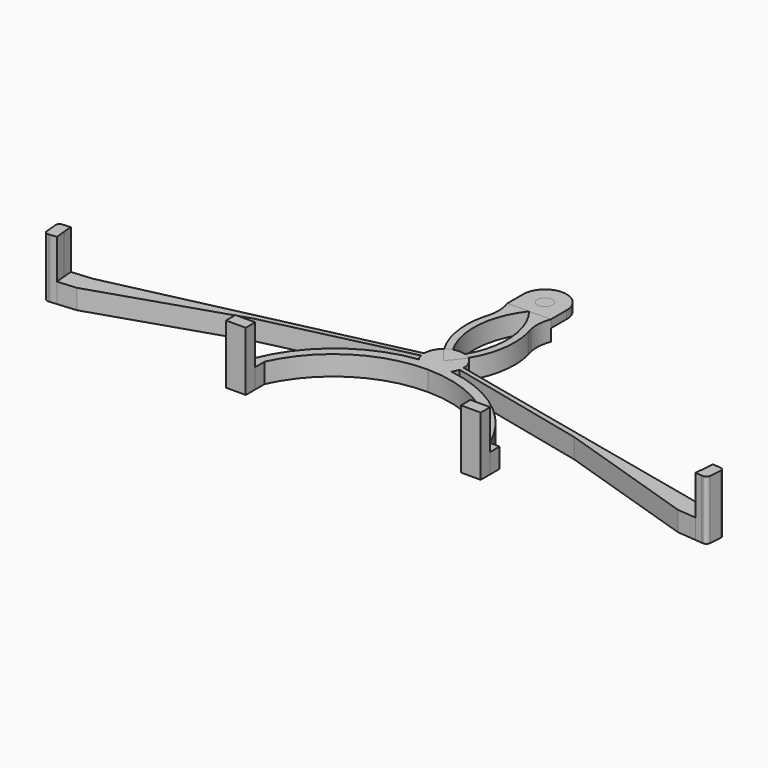
from build123d import *

# Parameters (mm, degrees)
F1_DEPTH = 15
F2_DEPTH = 5
F0_W     = 2.5
F0_H     = 3
F3_DEPTH = 5
F0_R     = 1.9
F4_DEPTH = 5
F5_DEPTH = 5
F6_DEPTH = 3


with BuildPart() as f1:
    # F0 (on Top) → F1 (new body)
    with BuildSketch(Plane.XY):
        with BuildLine():
            Line((-82.5, -21.5863350366), (-82.5, -16.5665013937))
            Line((-82.5, -16.5665013937), (-83.3699967597, -16.6440687753))
            ThreePointArc((-83.3699967597, -16.6440687753), (-84.0295454731, -16.9887980437), (-84.2521564375, -17.6989298148))
            Line((-84.2521564375, -17.6989298148), (-83.9808279356, -20.7421538184))
            ThreePointArc((-83.9808279356, -20.7421538184), (-83.6360986672, -21.4017025318), (-82.9259668961, -21.6243134962))
            Line((-82.9259668961, -21.6243134962), (-82.5, -21.5863350366))
        make_face()
        Polygon((-81.128345354, -18.9541238984), (-81.3503602858, -16.464001538), (-82.5, -16.5665013937), (-82.5, -21.5863350366), (-80.9063304222, -21.4442462589), align=None)
    extrude(amount=F1_DEPTH)


with BuildPart() as f1b:
    # F0 (on Top) → F1, piece 2 (new body)
    with BuildSketch(Plane.XY):
        with BuildLine():
            Line((83.3699963437, -16.6440687785), (82.5, -16.5665014329))
            Line((82.5, -16.5665014329), (82.5, -21.5863350764))
            Line((82.5, -21.5863350764), (82.9259664737, -21.6243134988))
            ThreePointArc((82.9259664737, -21.6243134988), (83.6360982451, -21.4017025353), (83.9808275143, -20.7421538224))
            Line((83.9808275143, -20.7421538224), (84.2521560202, -17.6989298191))
            ThreePointArc((84.2521560202, -17.6989298191), (84.0295450567, -16.9887980477), (83.3699963437, -16.6440687785))
        make_face()
        Polygon((82.5, -16.5665014329), (81.3503598701, -16.4640015386), (81.128344935, -18.9541238987), (80.90633, -21.4442462589), (82.5, -21.5863350764), align=None)
    extrude(amount=F1_DEPTH)


with BuildPart() as f1c:
    # F0 (on Top) → F1, piece 3 (new body)
    with BuildSketch(Plane.XY):
        Polygon((31.6213203436, -24.8786796564), (29.1213203436, -24.8786796564), (26.6213203436, -24.8786796564), (26.6213203436, -27.8786796564), (31.6213203436, -27.8786796564), align=None)
    extrude(amount=F1_DEPTH)


with BuildPart() as f1d:
    # F0 (on Top) → F1, piece 4 (new body)
    with BuildSketch(Plane.XY):
        Polygon((-29.8816396128, -25.5282291926), (-32.3816343716, -25.5231100091), (-32.3816343716, -28.5231100091), (-27.381644854, -28.5231100091), (-27.381644854, -25.5333483762), align=None)
    extrude(amount=F1_DEPTH)


with BuildPart() as f2:
    # F0 (on Top) → F2 (new body)
    with BuildSketch(Plane.XY):
        with BuildLine():
            Line((-2.1337940049, 27), (-5.5, 27))
            ThreePointArc((-5.5, 27), (-4.8940649659, 24.1020455305), (-5.1039532491, 21.1488702426))
            ThreePointArc((-5.1039532491, 21.1488702426), (-3.850388388, 24.1919569907), (-2.1337940049, 27))
        make_face()
        with BuildLine():
            Line((0, 27), (-2.1337940049, 27))
            ThreePointArc((-2.1337940049, 27), (-3.850388388, 24.1919569907), (-5.1039532491, 21.1488702426))
            ThreePointArc((-5.1039532491, 21.1488702426), (-5.278437838, 20.4458640026), (-5.5, 19.7562460986))
            ThreePointArc((-5.5, 19.7562460986), (-5.8710956961, 11.6043025747), (-3.0863215981, 3.9337792252))
            ThreePointArc((-3.0863215981, 3.9337792252), (-2.3467663768, 4.4150523862), (-1.5341266757, 4.7588291988))
            ThreePointArc((-1.5341266757, 4.7588291988), (-4.1864100938, 16.1152704866), (0, 27))
        make_face()
    extrude(amount=F2_DEPTH)


with BuildPart() as f2b:
    # F0 (on Top) → F2, piece 2 (new body)
    with BuildSketch(Plane.XY):
        with BuildLine():
            Line((2.1337940049, 27), (0, 27))
            ThreePointArc((0, 27), (4.1765920633, 16.1147529743), (1.5306162106, 4.7599594553))
            ThreePointArc((1.5306162106, 4.7599594553), (2.3451379758, 4.4159175575), (3.0863215981, 3.9337792252))
            ThreePointArc((3.0863215981, 3.9337792252), (5.8710956961, 11.6043025747), (5.5, 19.7562460986))
            ThreePointArc((5.5, 19.7562460986), (5.2493596136, 20.5144731098), (5.0579844363, 21.289782303))
            ThreePointArc((5.0579844363, 21.289782303), (3.8167255549, 24.2579809722), (2.1337940049, 27))
        make_face()
        with BuildLine():
            Line((5.5, 27), (2.1337940049, 27))
            ThreePointArc((2.1337940049, 27), (3.8167255549, 24.2579809722), (5.0579844363, 21.289782303))
            ThreePointArc((5.0579844363, 21.289782303), (4.8757325261, 24.1761066094), (5.5, 27))
        make_face()
    extrude(amount=F2_DEPTH)


with BuildPart() as f2c:
    # F0 (on Top) → F2, piece 3 (new body)
    with BuildSketch(Plane.XY):
        with BuildLine():
            ThreePointArc((0, 0), (-1.6614515986, 1.8740823074), (-3.0863215981, 3.9337792252))
            ThreePointArc((-3.0863215981, 3.9337792252), (-4.4961988385, 2.1872805043), (-5, 0))
            Line((-5, 0), (0, 0))
        make_face()
        with BuildLine():
            ThreePointArc((5, 0), (4.4961988385, 2.1872805043), (3.0863215981, 3.9337792252))
            ThreePointArc((3.0863215981, 3.9337792252), (1.6614515986, 1.8740823074), (0, 0))
            Line((0, 0), (5, 0))
        make_face()
        with BuildLine():
            Line((0, 0), (-5, 0))
            ThreePointArc((-5, 0), (-4.9671130397, -0.5725277732), (-4.8688847796, -1.137524067))
            Line((-4.8688847796, -1.137524067), (0, 0))
        make_face()
        with BuildLine():
            ThreePointArc((-4.8688847796, -1.137524067), (-4.9671130397, -0.5725277732), (-5, 0))
            Line((-5, 0), (-76.1126271301, -15.9970144582))
            Line((-76.1126271301, -15.9970144582), (-76.1126271301, -17.7822949373))
            Line((-76.1126271301, -17.7822949373), (-40.564172677, -9.4770619492))
            Line((-40.564172677, -9.4770619492), (-4.8688847796, -1.137524067))
        make_face()
        with BuildLine():
            Line((5, 0), (0, 0))
            Line((0, 0), (4.8688847783, -1.1375240726))
            ThreePointArc((4.8688847783, -1.1375240726), (4.9671130394, -0.572527776), (5, 0))
        make_face()
        with BuildLine():
            Line((0, -2.5), (0, 0))
            Line((0, 0), (-4.8688847796, -1.137524067))
            ThreePointArc((-4.8688847796, -1.137524067), (-4.5953849074, -1.9703902031), (-4.1806287521, -2.7426890522))
            ThreePointArc((-4.1806287521, -2.7426890522), (-2.0942964003, -2.5527490751), (0, -2.5))
        make_face()
        with BuildLine():
            Line((4.8688847783, -1.1375240726), (0, 0))
            Line((0, 0), (0, -2.5))
            ThreePointArc((0, -2.5), (2.0756234829, -2.5833806697), (4.1414358733, -2.8015190356))
            ThreePointArc((4.1414358733, -2.8015190356), (4.5813414379, -2.0028256613), (4.8688847783, -1.1375240726))
        make_face()
        with BuildLine():
            Line((76.1126265372, -15.9970144361), (5, 0))
            ThreePointArc((5, 0), (4.9671130394, -0.572527776), (4.8688847783, -1.1375240726))
            Line((4.8688847783, -1.1375240726), (40.5641724675, -9.4770619494))
            Line((40.5641724675, -9.4770619494), (76.1126265372, -17.7822948909))
            Line((76.1126265372, -17.7822948909), (76.1126265372, -15.9970144361))
        make_face()
        Polygon((-76.1126271301, -17.7822949373), (-76.1126271301, -15.9970144582), (-81.3503602858, -16.464001538), (-81.128345354, -18.9541238984), align=None)
        with BuildLine():
            ThreePointArc((4.1414358733, -2.8015190356), (2.0756234829, -2.5833806697), (0, -2.5))
            Line((0, -2.5), (0, -5))
            ThreePointArc((0, -5), (2.3443980914, -4.4163104045), (4.1414358733, -2.8015190356))
        make_face()
        with BuildLine():
            Line((0, -5), (0, -2.5))
            ThreePointArc((0, -2.5), (-2.0942964003, -2.5527490751), (-4.1806287521, -2.7426890522))
            ThreePointArc((-4.1806287521, -2.7426890522), (-2.4045705015, -4.3838385809), (-0.0660587142, -4.9995636056))
            ThreePointArc((-0.0660587142, -4.9995636056), (-0.0330300778, -4.9998909002), (0, -5))
        make_face()
        Polygon((81.3503598701, -16.4640015386), (76.1126265372, -15.9970144361), (76.1126265372, -17.7822948909), (81.128344935, -18.9541238987), align=None)
        with BuildLine():
            ThreePointArc((-0.0660587142, -4.9995636056), (-2.4045705015, -4.3838385809), (-4.1806287521, -2.7426890522))
            ThreePointArc((-4.1806287521, -2.7426890522), (-19.7252165616, -9.1292774686), (-29.8754860972, -22.5231100091))
            Line((-29.8754860972, -22.5231100091), (-27.381644854, -22.5231100091))
            ThreePointArc((-27.381644854, -22.5231100091), (-16.318878423, -9.7162267561), (-0.0660587142, -4.9995636056))
        make_face()
        Polygon((-76.1126271301, -21.0168481011), (-40.564172677, -9.4770619492), (-76.1126271301, -17.7822949373), align=None)
        Polygon((-76.1126271301, -21.0168481011), (-76.1126271301, -17.7822949373), (-81.128345354, -18.9541238984), (-80.9063304222, -21.4442462589), align=None)
        with BuildLine():
            ThreePointArc((29.1213203436, -21.8786796564), (19.1406778811, -9.0543892937), (4.1414358733, -2.8015190356))
            ThreePointArc((4.1414358733, -2.8015190356), (2.3443980914, -4.4163104045), (0, -5))
            ThreePointArc((0, -5), (15.7253308616, -9.6308830492), (26.6213203436, -21.8786796564))
            Line((26.6213203436, -21.8786796564), (29.1213203436, -21.8786796564))
        make_face()
        Polygon((76.1126265372, -17.7822948909), (40.5641724675, -9.4770619494), (76.1126265372, -21.0168480796), align=None)
        Polygon((81.128344935, -18.9541238987), (76.1126265372, -17.7822948909), (76.1126265372, -21.0168480796), (80.90633, -21.4442462589), align=None)
        Polygon((-29.8816291304, -25.5231100091), (-29.8754860972, -22.5231100091), (-32.3816343716, -22.5231100091), (-32.3816343716, -25.5231100091), align=None)
        Polygon((-27.381644854, -22.5231100091), (-29.8754860972, -22.5231100091), (-29.8816291304, -25.5231100091), (-27.381644854, -25.5231100091), align=None)
        with Locations((27.8713203436, -23.3786796564)):
            Rectangle(F0_W, F0_H)
        with Locations((30.3713203436, -23.3786796564)):
            Rectangle(F0_W, F0_H)
    extrude(amount=F2_DEPTH)


with BuildPart() as f3:
    # F0 (on Top) → F3 (new body)
    with BuildSketch(Plane.XY):
        with BuildLine():
            ThreePointArc((0, 2.5), (0.8041462109, 3.6036756124), (1.5306162106, 4.7599594553))
            ThreePointArc((1.5306162106, 4.7599594553), (-0.0018439661, 4.99999966), (-1.5341266757, 4.7588291988))
            ThreePointArc((-1.5341266757, 4.7588291988), (-0.8059688668, 3.6029911718), (0, 2.5))
        make_face()
        with BuildLine():
            ThreePointArc((3.0863215981, 3.9337792252), (2.3451379758, 4.4159175575), (1.5306162106, 4.7599594553))
            ThreePointArc((1.5306162106, 4.7599594553), (0.8041462109, 3.6036756124), (0, 2.5))
            ThreePointArc((0, 2.5), (-0.8059688668, 3.6029911718), (-1.5341266757, 4.7588291988))
            ThreePointArc((-1.5341266757, 4.7588291988), (-2.3467663768, 4.4150523862), (-3.0863215981, 3.9337792252))
            ThreePointArc((-3.0863215981, 3.9337792252), (-1.6614515986, 1.8740823074), (0, 0))
            ThreePointArc((0, 0), (1.6614515986, 1.8740823074), (3.0863215981, 3.9337792252))
        make_face()
    extrude(amount=F3_DEPTH)


with BuildPart() as f4:
    # F0 (on Top) → F4 (new body)
    with BuildSketch(Plane.XY):
        with Locations((0, 32)):
            Circle(F0_R)
    extrude(amount=F4_DEPTH)


with BuildPart() as f5:
    # F0 (on Top) → F5 (new body)
    with BuildSketch(Plane.XY):
        with BuildLine():
            Line((-5.5, 32), (-5.5, 27))
            Line((-5.5, 27), (-2.1337940049, 27))
            ThreePointArc((-2.1337940049, 27), (-1.1162134987, 28.2920924976), (0, 29.5))
            ThreePointArc((0, 29.5), (1.1162134987, 28.2920924976), (2.1337940049, 27))
            Line((2.1337940049, 27), (5.5, 27))
            Line((5.5, 27), (5.5, 32))
            ThreePointArc((5.5, 32), (0, 37.5), (-5.5, 32))
        make_face()
        with Locations((0, 32)):
            Circle(F0_R, mode=Mode.SUBTRACT)
        with BuildLine():
            ThreePointArc((0, 29.5), (-1.1162134987, 28.2920924976), (-2.1337940049, 27))
            Line((-2.1337940049, 27), (0, 27))
            Line((0, 27), (2.1337940049, 27))
            ThreePointArc((2.1337940049, 27), (1.1162134987, 28.2920924976), (0, 29.5))
        make_face()
    extrude(amount=F5_DEPTH)

    # F0 (on Top) → F6 (cut)
    with BuildSketch(Plane.XY):
        with BuildLine():
            Line((-5.5, 32), (-5.5, 27))
            Line((-5.5, 27), (-2.1337940049, 27))
            ThreePointArc((-2.1337940049, 27), (-1.1162134987, 28.2920924976), (0, 29.5))
            ThreePointArc((0, 29.5), (1.1162134987, 28.2920924976), (2.1337940049, 27))
            Line((2.1337940049, 27), (5.5, 27))
            Line((5.5, 27), (5.5, 32))
            ThreePointArc((5.5, 32), (0, 37.5), (-5.5, 32))
        make_face()
        with Locations((0, 32)):
            Circle(F0_R, mode=Mode.SUBTRACT)
        with BuildLine():
            ThreePointArc((0, 29.5), (-1.1162134987, 28.2920924976), (-2.1337940049, 27))
            Line((-2.1337940049, 27), (0, 27))
            Line((0, 27), (2.1337940049, 27))
            ThreePointArc((2.1337940049, 27), (1.1162134987, 28.2920924976), (0, 29.5))
        make_face()
    extrude(amount=F6_DEPTH, mode=Mode.SUBTRACT)


solid = Compound([f1.part, f1b.part, f1c.part, f1d.part, f2.part, f2b.part, f2c.part, f3.part, f4.part, f5.part])
